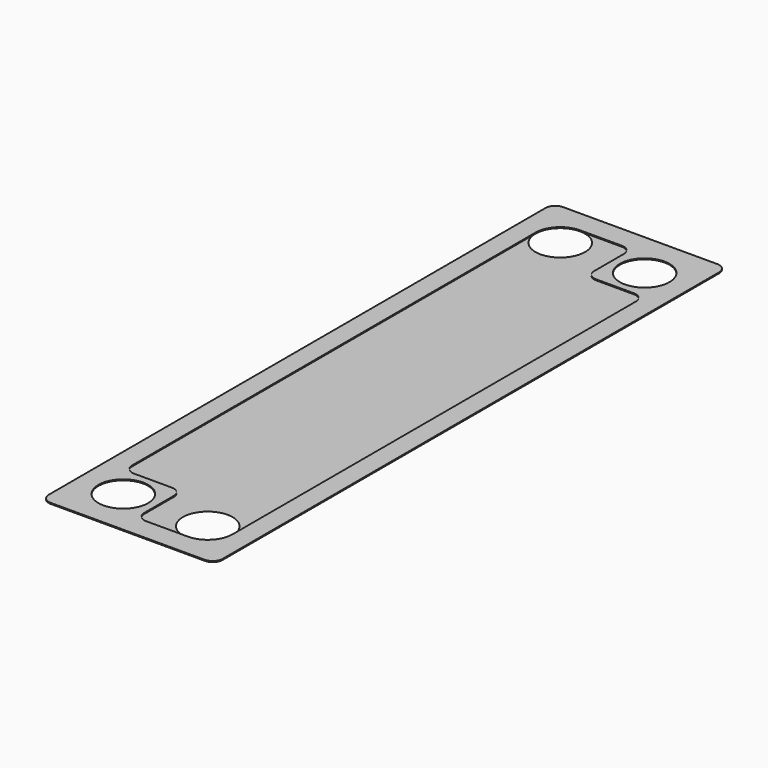
from build123d import *

# Parameters (mm, degrees)
F0_W     = 88.9
F0_H     = 327.66
F0_R     = 12.7
F1_DEPTH = 0.5
F2_DEPTH = 0.005
F3_R     = 5.08


# Not quite as in the source:
# - a feature names something its author has since deleted; it is built from what else it names


with BuildPart() as f1:
    # F0 (on Top) → F1 (new body)
    with BuildSketch(Plane.XY):
        Rectangle(F0_W, F0_H)
        with Locations((-21.59, -139.7)):
            Circle(F0_R, mode=Mode.SUBTRACT)
        with BuildLine():
            ThreePointArc((-34.29, 139.7), (-30.5702561211, 148.6802561211), (-21.59, 152.4))
            Line((-21.59, 152.4), (4.826, 152.4))
            Line((4.826, 152.4), (4.826, 123.2959434))
            Line((4.826, 123.2959434), (34.29, 123.2959434))
            Line((34.29, 123.2959434), (34.29, -139.7))
            ThreePointArc((34.29, -139.7), (30.5702561211, -148.6802561211), (21.59, -152.4))
            Line((21.59, -152.4), (-4.826, -152.4))
            Line((-4.826, -152.4), (-4.826, -123.2959434))
            Line((-4.826, -123.2959434), (-34.29, -123.2959434))
            Line((-34.29, -123.2959434), (-34.29, 139.7))
        make_face(mode=Mode.SUBTRACT)
        with Locations((21.59, 139.7)):
            Circle(F0_R, mode=Mode.SUBTRACT)
    extrude(amount=F1_DEPTH)

    # F0 (on Top) → F2 (join)
    with BuildSketch(Plane.XY):
        with BuildLine():
            ThreePointArc((-21.59, 152.4), (-12.6097438789, 148.6802561211), (-8.89, 139.7))
            ThreePointArc((-8.89, 139.7), (-21.59, 127), (-34.29, 139.7))
            Line((-34.29, 139.7), (-34.29, -123.2959434))
            Line((-34.29, -123.2959434), (-4.826, -123.2959434))
            Line((-4.826, -123.2959434), (-4.826, -152.4))
            Line((-4.826, -152.4), (21.59, -152.4))
            ThreePointArc((21.59, -152.4), (12.6097438789, -130.7197438789), (34.29, -139.7))
            Line((34.29, -139.7), (34.29, 123.2959434))
            Line((34.29, 123.2959434), (4.826, 123.2959434))
            Line((4.826, 123.2959434), (4.826, 152.4))
            Line((4.826, 152.4), (-21.59, 152.4))
        make_face()
    extrude(amount=F2_DEPTH)

    # F3
    f3_edges = [f1.edges().sort_by_distance(p)[0] for p in [
        (-44.45, 163.83, 0.25),
        (44.45, -163.83, 0.25),
        (-44.45, -163.83, 0.25),
        (44.45, 163.83, 0.25),
        (4.826, 152.4, 0.2525),
        (4.826, 123.295943, 0.2525),
        (34.29, 123.295943, 0.2525),
        (-4.826, -152.4, 0.2525),
        (-4.826, -123.295943, 0.2525),
        (-34.29, -123.295943, 0.2525),
    ]]
    fillet(f3_edges, radius=F3_R)


solid = f1.part
